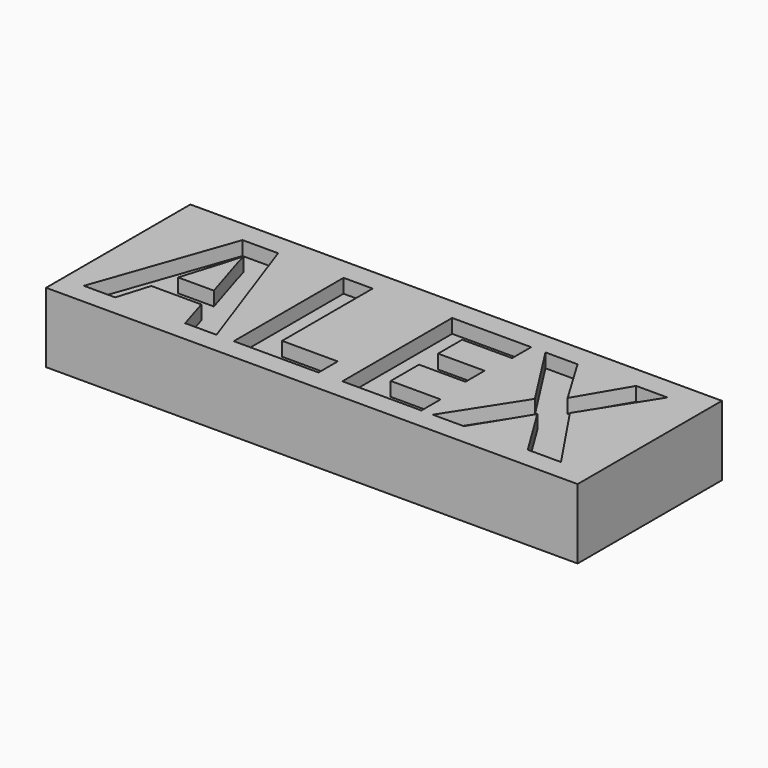
from build123d import *

# Parameters (mm, degrees)
F1_W         = 76
F1_H         = 25.7889570552
F2_DEPTH     = 10
F0_TEXT_SIZE = 27.4846625767
F3_DEPTH     = 2


# Not quite as in the source:
# - Text() gives the source's letters only with a copy of the font that has no kerning and outlines rounded to 1/6400 em; it was checked with that copy


with BuildPart() as f2:
    # F1 (on Top) → F2 (new body)
    with BuildSketch(Plane.XY):
        Rectangle(F1_W, F1_H)
    extrude(amount=-F2_DEPTH)

    # F0 (on Top) → F3 (cut)
    with BuildSketch(Plane.XY):
        with Locations((-35, -9.8944785276)):
            Text('ALEX', F0_TEXT_SIZE, font='Open Sans', font_style=FontStyle.BOLD, text_align=(TextAlign.LEFT, TextAlign.BOTTOM))
    extrude(amount=-F3_DEPTH, mode=Mode.SUBTRACT)


solid = f2.part
